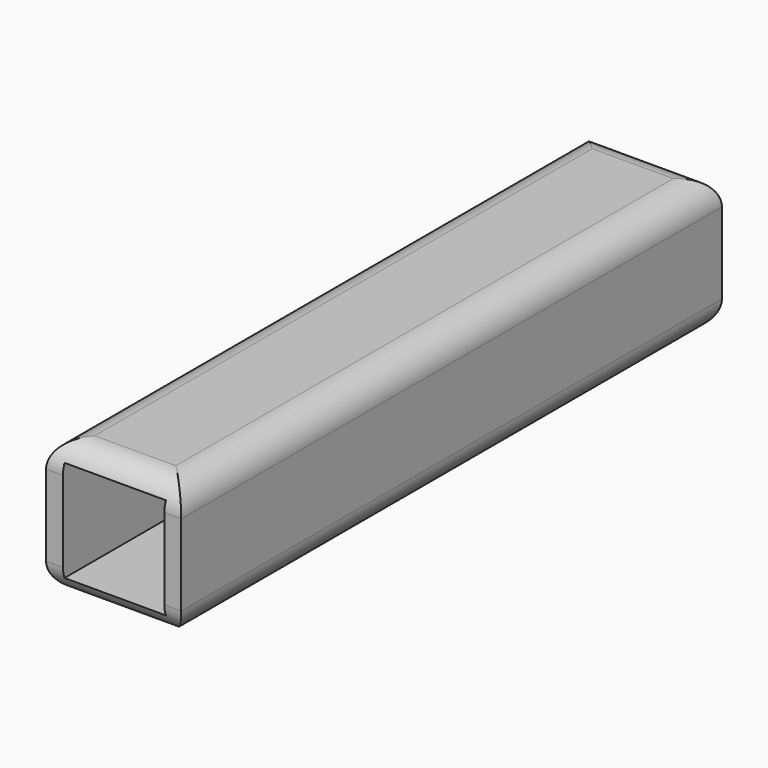
from build123d import *

# Parameters (mm, degrees)
F0_W        = 25.4
F0_H        = 25.4
F0_W_2      = 19.05
F0_H_2      = 19.05
F1_DEPTH    = 127
F2_T1_DEPTH = 152.4
F2_T3_DEPTH = 50.8


# Not quite as in the source:
# - a fillet or chamfer that OpenCascade refuses, or shapes differently, is made with other operations: its cross-section is extruded or revolved along the edge and cut away or added


with BuildPart() as f1:
    # F0 (on Front) → F1 (new body)
    with BuildSketch(Plane.XZ):
        Rectangle(F0_W, F0_H)
        Rectangle(F0_W_2, F0_H_2, mode=Mode.SUBTRACT)
    extrude(amount=F1_DEPTH)

    # F2: fillet of radius 5.08 on 8 edges, made by hand

    # F2_s2 → F2_t1 (cut)
    with BuildSketch(Plane.XZ.offset(-12.7)):
        with BuildLine():
            ThreePointArc((12.7, 7.62), (11.2121024484, 11.2121024484), (7.62, 12.7))
            Line((7.62, 12.7), (12.7, 12.7))
            Line((12.7, 12.7), (12.7, 7.62))
        make_face()
        with BuildLine():
            ThreePointArc((-12.7, 7.62), (-11.2121024484, 11.2121024484), (-7.62, 12.7))
            Line((-7.62, 12.7), (-12.7, 12.7))
            Line((-12.7, 12.7), (-12.7, 7.62))
        make_face()
        with BuildLine():
            ThreePointArc((-12.7, -7.62), (-11.2121024484, -11.2121024484), (-7.62, -12.7))
            Line((-7.62, -12.7), (-12.7, -12.7))
            Line((-12.7, -12.7), (-12.7, -7.62))
        make_face()
        with BuildLine():
            ThreePointArc((7.62, -12.7), (11.2121024484, -11.2121024484), (12.7, -7.62))
            Line((12.7, -7.62), (12.7, -12.7))
            Line((12.7, -12.7), (7.62, -12.7))
        make_face()
    extrude(amount=F2_T1_DEPTH, mode=Mode.SUBTRACT)

    # F2_s4 → F2_t3 (cut)
    with BuildSketch(Plane.YZ.offset(-25.4)):
        with BuildLine():
            ThreePointArc((-5.08, 12.7), (-1.4878975516, 11.2121024484), (0, 7.62))
            Line((0, 7.62), (0, 12.7))
            Line((0, 12.7), (-5.08, 12.7))
        make_face()
        with BuildLine():
            ThreePointArc((-121.92, 12.7), (-125.5121024484, 11.2121024484), (-127, 7.62))
            Line((-127, 7.62), (-127, 12.7))
            Line((-127, 12.7), (-121.92, 12.7))
        make_face()
        with BuildLine():
            ThreePointArc((-5.08, -12.7), (-1.4878975516, -11.2121024484), (0, -7.62))
            Line((0, -7.62), (0, -12.7))
            Line((0, -12.7), (-5.08, -12.7))
        make_face()
        with BuildLine():
            ThreePointArc((-121.92, -12.7), (-125.5121024484, -11.2121024484), (-127, -7.62))
            Line((-127, -7.62), (-127, -12.7))
            Line((-127, -12.7), (-121.92, -12.7))
        make_face()
    extrude(amount=F2_T3_DEPTH, mode=Mode.SUBTRACT)


solid = f1.part
